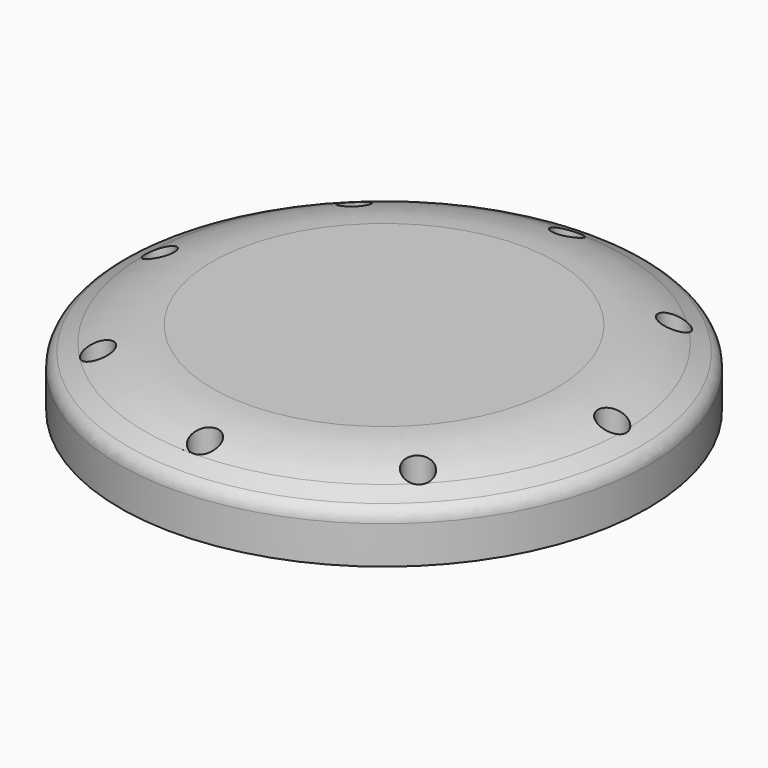
from build123d import *

# Parameters (mm, degrees)
F0_R     = 88.9
F1_DEPTH = 25.4
F2_R     = 4.7625
F3_DEPTH = 25.401
F6_R     = 5.08


# Not quite as in the source:
# - a fillet or chamfer that OpenCascade refuses, or shapes differently, is made with other operations: its cross-section is extruded or revolved along the edge and cut away or added


with BuildPart() as f1:
    # F0 (on Top) → F1 (new body)
    with BuildSketch(Plane.XY):
        with Locations((-0.2919610997, -0.4379486491)):
            Circle(F0_R)
    extrude(amount=F1_DEPTH)

    # F2 (on face) → F3 (cut, through all)
    with BuildSketch(Plane.XY.offset(25.4)):
        with Locations((76.2, 0)):
            Circle(F2_R)
        with Locations((53.8815367264, 53.8815367264)):
            Circle(F2_R)
        with Locations((0, 76.2)):
            Circle(F2_R)
        with Locations((-53.8815367264, 53.8815367264)):
            Circle(F2_R)
        with Locations((-76.2, 0)):
            Circle(F2_R)
        with Locations((-53.8815367264, -53.8815367264)):
            Circle(F2_R)
        with Locations((0, -76.2)):
            Circle(F2_R)
        with Locations((53.8815367264, -53.8815367264)):
            Circle(F2_R)
    extrude(amount=-F3_DEPTH, mode=Mode.SUBTRACT)

    # F4: chamfer of 19.05 x 9.525 on 1 edges, made by hand

    # F4_s1 → F4_t2 (revolve, cut)
    with BuildSketch(Plane.XZ.offset(0.4379486491)):
        Polygon((88.6080389003, 15.875), (69.5580389003, 25.4), (88.6080389003, 25.4), align=None)
    revolve(axis=Axis((-0.2919610997, -0.4379486491, 25.4), (0, 0, 1)), mode=Mode.SUBTRACT)

    # F5: fillet of radius 50.8 on 1 edges, made by hand

    # F5_s1 → F5_t2 (revolve, cut)
    with BuildSketch(Plane.XZ.offset(0.4379486491)):
        with BuildLine():
            ThreePointArc((80.2842362947, 20.0369013028), (69.2372340071, 24.041048665), (57.5657856433, 25.4))
            Line((57.5657856433, 25.4), (69.5580389003, 25.4))
            Line((69.5580389003, 25.4), (80.2842362947, 20.0369013028))
        make_face()
    revolve(axis=Axis((-0.2919610997, -0.4379486491, 25.4), (0, 0, 1)), mode=Mode.SUBTRACT)

    # F6
    f6_edges = [f1.edges().sort_by_distance(p)[0] for p in [
        (-89.191961, -0.437949, 15.875),
    ]]
    fillet(f6_edges, radius=F6_R)


solid = f1.part
